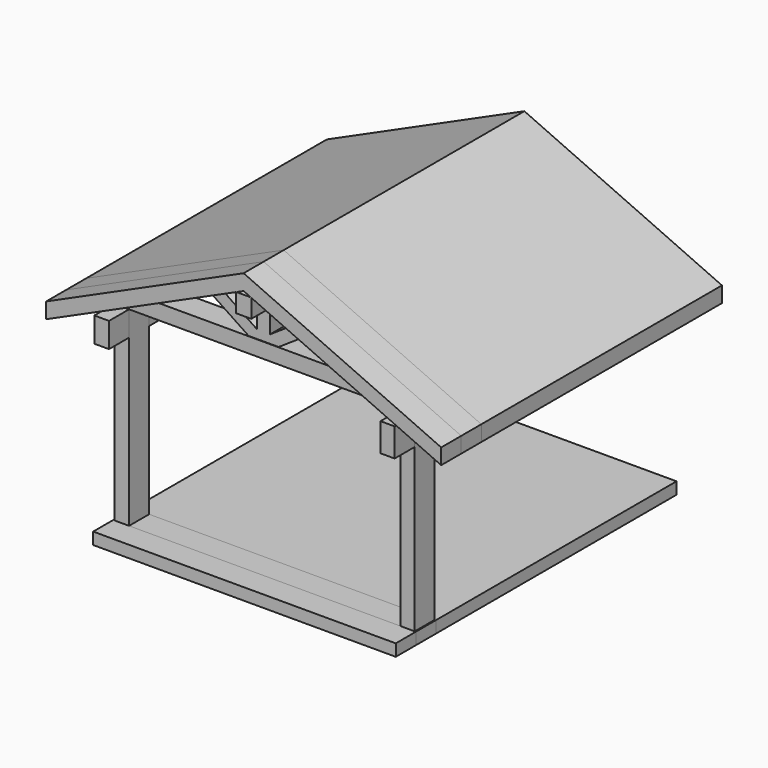
from build123d import *

# Parameters (mm, degrees)
F2_DEPTH      = 25.4
F2_DEPTH_BACK = 152.4
F0_W          = 7.4506402016
F0_H          = 12.6087740064
F0_W_2        = 7.1640759706
F0_H_2        = 14.3281519413
F1_W          = 7.7642686665
F1_H          = 9.5112249255
F0_H_3        = 83.9629881084
F3_DEPTH      = 12.7
F6_DEPTH      = 12.7
F4_W          = 5.8232028969
F4_H          = 12.3464902455
F10_DEPTH     = 12.7


# Not quite as in the source:
# - ends of sketch curves that miss each other by under 0.0002 mm in the source are joined


with BuildPart() as f2:
    # F0 (on Front) → F2 (new body, two sides)
    with BuildSketch(Plane.XZ) as f2_sk:
        Polygon((-75.6526514888, 47.9380041004), (-75.6526514888, 41.6479729853), (-61.7104200599, 47.9380041004), align=None)
        Polygon((61.7104200599, 47.9380041004), (76.5123516321, 41.2601196722), (76.5123516321, 47.9380041004), align=None)
        Polygon((-100.0904308233, 30.6228803963), (-75.6526514888, 41.6479729853), (-75.6526514888, 47.9380041004), (-61.7104200599, 47.9380041004), (-35.0340465252, 59.973037404), (-27.9464338127, 63.1706105272), (-3.864014828, 74.0353824624), (0, 75.7786309245), (0, 83.7069652426), (-100.0904308233, 38.5512147144), align=None)
        Polygon((76.5123516321, 47.9380041004), (76.5123516321, 41.2601196722), (100.0904308233, 30.6228803963), (100.0904308233, 38.5512147144), (0, 83.7069652426), (0, 75.7786309245), (3.864014828, 74.0353824624), (27.9464338127, 63.1706105272), (35.0340465252, 59.973037404), (61.7104200599, 47.9380041004), align=None)
    extrude(amount=F2_DEPTH)
    extrude(f2_sk.sketch, amount=-F2_DEPTH_BACK)


with BuildPart() as f2b:
    # F0 (on Front) → F2, piece 2 (new body, two sides)
    with BuildSketch(Plane.XZ) as f2_2_sk:
        Polygon((-75.6526514888, -56.3096441329), (-76.2257799506, -56.3096441329), (-76.2257799506, -62.3274669051), (77.085480094, -62.3274669051), (77.085480094, -56.3096441329), (76.5123516321, -56.3096441329), (69.3482756615, -56.3096441329), (-68.2020112872, -56.3096441329), align=None)
    extrude(amount=F2_DEPTH)
    extrude(f2_2_sk.sketch, amount=-F2_DEPTH_BACK)


with BuildPart() as f2c:
    # F0 (on Front) → F2, piece 3 (new body, two sides)
    with BuildSketch(Plane.XZ) as f2_3_sk:
        with Locations((-71.927331388, 33.9577309787)):
            Rectangle(F0_W, F0_H)
    extrude(amount=F2_DEPTH)
    extrude(f2_3_sk.sketch, amount=-F2_DEPTH_BACK)


with BuildPart() as f2d:
    # F0 (on Front) → F2, piece 4 (new body, two sides)
    with BuildSketch(Plane.XZ) as f2_4_sk:
        with Locations((72.9303136468, 33.0980420113)):
            Rectangle(F0_W_2, F0_H_2)
    extrude(amount=F2_DEPTH)
    extrude(f2_4_sk.sketch, amount=-F2_DEPTH_BACK)


with BuildPart() as f2e:
    # F1 (on Front) → F2, piece 5 (new body, two sides)
    with BuildSketch(Plane.XZ) as f2_5_sk:
        with Locations((2.328e-07, 69.3615563214)):
            Rectangle(F1_W, F1_H)
    extrude(amount=F2_DEPTH)
    extrude(f2_5_sk.sketch, amount=-F2_DEPTH_BACK)


with BuildPart() as f3:
    # F0 (on Front) → F3 (new body)
    with BuildSketch(Plane.XZ):
        Polygon((-75.6526514888, -56.3096441329), (-76.2257799506, -56.3096441329), (-76.2257799506, -62.3274669051), (77.085480094, -62.3274669051), (77.085480094, -56.3096441329), (76.5123516321, -56.3096441329), (69.3482756615, -56.3096441329), (-68.2020112872, -56.3096441329), align=None)
        with Locations((-71.927331388, -14.3281500787)):
            Rectangle(F0_W, F0_H_3)
        with Locations((-71.927331388, 33.9577309787)):
            Rectangle(F0_W, F0_H)
        Polygon((69.3482756615, 25.9339660406), (69.3482756615, -56.3096422702), (76.5123516321, -56.3096441329), (76.5123516321, 25.9339660406), align=None)
        Polygon((-75.6526514888, 41.6479729853), (-75.6526514888, 40.2621179819), (-68.2020112872, 40.2621179819), (69.3482756615, 40.2621179819), (76.5123516321, 40.2621179819), (76.5123516321, 41.2601196722), (61.7104200599, 47.9380041004), (10.3307002624, 47.9380041004), (3.864014828, 47.9380041004), (-3.864014828, 47.9380041004), (-10.3307002624, 47.9380041004), (-61.7104200599, 47.9380041004), align=None)
        with Locations((72.9303136468, 33.0980420113)):
            Rectangle(F0_W_2, F0_H_2)
        Polygon((-100.0904308233, 30.6228803963), (-75.6526514888, 41.6479729853), (-75.6526514888, 47.9380041004), (-61.7104200599, 47.9380041004), (-35.0340465252, 59.973037404), (-27.9464338127, 63.1706105272), (-3.864014828, 74.0353824624), (0, 75.7786309245), (0, 83.7069652426), (-100.0904308233, 38.5512147144), align=None)
        Polygon((-75.6526514888, 47.9380041004), (-75.6526514888, 41.6479729853), (-61.7104200599, 47.9380041004), align=None)
        Polygon((61.7104200599, 47.9380041004), (76.5123516321, 41.2601196722), (76.5123516321, 47.9380041004), align=None)
        Polygon((76.5123516321, 47.9380041004), (76.5123516321, 41.2601196722), (100.0904308233, 30.6228803963), (100.0904308233, 38.5512147144), (0, 83.7069652426), (0, 75.7786309245), (3.864014828, 74.0353824624), (27.9464338127, 63.1706105272), (35.0340465252, 59.973037404), (61.7104200599, 47.9380041004), align=None)
    extrude(amount=F3_DEPTH)


with BuildPart() as f6:
    # F5 (on face) → F6 (new body)
    with BuildSketch(Plane.XZ):
        Polygon((3.6880273838, 55.2862646402), (2.8213392943, 54.8919215798), (2.8213392943, 48.1377206743), (3.6880273838, 48.5300727755), (3.6880273838, 54.9006089568), align=None)
        Polygon((2.8213392943, 61.1069290045), (2.8213392943, 54.8919215798), (3.6880273838, 55.2862646402), (3.6880273838, 61.1069290045), align=None)
        Polygon((2.8213392943, 48.1377206743), (2.8213392943, 54.8919215798), (2.8213392943, 61.1069290045), (-2.8213392943, 61.1069290045), (-3.6880273838, 61.1069290045), (-3.6880273838, 54.9006089568), (-3.6880273838, 48.1377206743), align=None)
        Polygon((24.6090814471, 64.8053437471), (3.6880273838, 55.2862646402), (3.6880273838, 54.9006089568), (3.6880273838, 48.5300727755), (31.4697353526, 61.1069290045), align=None)
        Polygon((-2.8213392943, 61.1069290045), (2.8213392943, 61.1069290045), (2.8213392943, 73.9230662584), (0, 74.0071956538), (-3.6880273838, 74.1171687841), (-3.6880273838, 61.1069290045), align=None)
        Polygon((2.8213392943, 73.9230662584), (2.8213392943, 61.1069290045), (3.6880273838, 61.1069290045), (3.6880273838, 74.1171687841), (0, 74.0071956538), align=None)
        Polygon((-3.6880273838, 48.1068715453), (-3.6880273838, 48.1377206743), (-3.6880273838, 54.9006089568), (-24.8206017808, 64.4673839815), (-32.4158221483, 61.11202389), align=None)
    extrude(amount=F6_DEPTH)


with BuildPart() as f6b:
    # F4 (on Front) → F6, piece 2 (new body)
    with BuildSketch(Plane.XZ):
        with Locations((0, 67.707815617)):
            Rectangle(F4_W, F4_H)
    extrude(amount=F6_DEPTH)


with BuildPart() as f10:
    # F9 (on Front) → F10 (new body)
    with BuildSketch(Plane.XZ):
        Polygon((-7.5701624155, 48.1068715453), (-3.2998144161, 48.1068715453), (-3.2998144161, 52.3772165179), (-22.6707686226, 65.3488352822), (-29.3101165444, 62.664873898), align=None)
        Polygon((-3.2998144161, 52.3772165179), (-3.2998144161, 48.1068715453), (3.2998144161, 48.1068715453), (3.2998144161, 52.3772165179), (3.2998144161, 65.5764713883), (-3.2998144161, 65.5764713883), align=None)
        Polygon((3.2998144161, 52.3772165179), (3.2998144161, 48.1068715453), (7.5701624155, 48.1068715453), (29.3101165444, 62.664873898), (22.6707686226, 65.3488352822), align=None)
        Polygon((-3.2998144161, 74.1617158055), (-3.2998144161, 65.5764713883), (3.2998144161, 65.5764713883), (3.2998144161, 74.1617158055), (0, 75.7939517498), align=None)
    extrude(amount=F10_DEPTH)


solid = Compound([f2.part, f2b.part, f2c.part, f2d.part, f2e.part, f3.part, f10.part])
